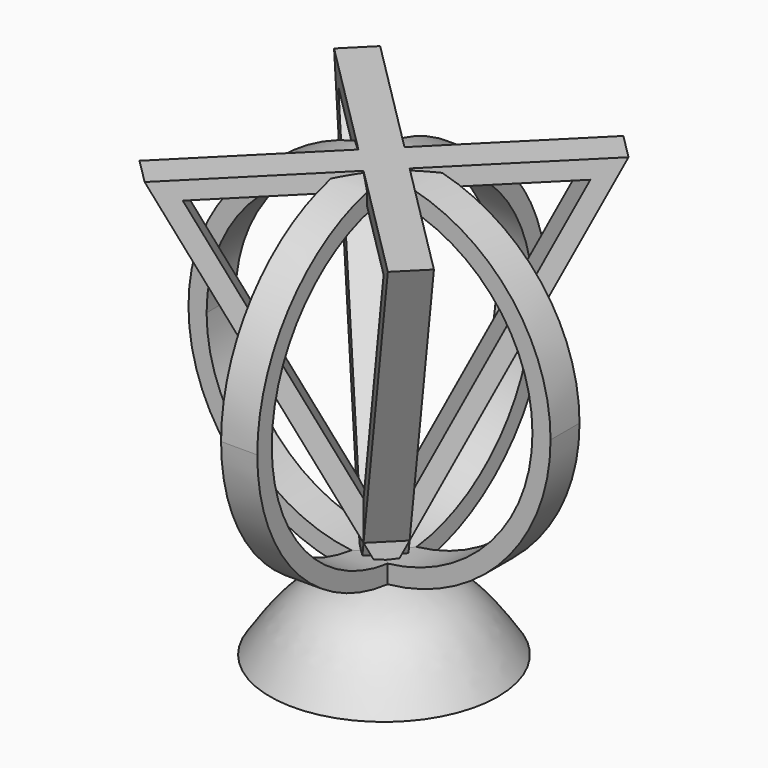
from build123d import *

# Parameters (mm, degrees)
F1_DEPTH = 5.08
F2_DEPTH = 5.08
F3_COUNT = 4
F6_DEPTH = 5.08
F7_DEPTH = 5.08
F8_COUNT = 4


with BuildPart() as f1:
    # F0 (on Front) → F1 (new body)
    with BuildSketch(Plane.XZ):
        with BuildLine():
            ThreePointArc((0, 45.72), (32.328922, 32.328922), (45.72, 0))
            ThreePointArc((45.72, 0), (32.328922, -32.328922), (0, -45.72))
            Line((0, -45.72), (0, -50.8))
            ThreePointArc((0, -50.8), (35.921024, -35.921024), (50.8, 0))
            ThreePointArc((50.8, 0), (35.921024, 35.921024), (0, 50.8))
            Line((0, 50.8), (0, 45.72))
        make_face()
    extrude(amount=F1_DEPTH)

    # F0 (on Front) → F2 (join)
    with BuildSketch(Plane.XZ):
        with BuildLine():
            ThreePointArc((0, 45.72), (32.328922, 32.328922), (45.72, 0))
            ThreePointArc((45.72, 0), (32.328922, -32.328922), (0, -45.72))
            Line((0, -45.72), (0, -50.8))
            ThreePointArc((0, -50.8), (35.921024, -35.921024), (50.8, 0))
            ThreePointArc((50.8, 0), (35.921024, 35.921024), (0, 50.8))
            Line((0, 50.8), (0, 45.72))
        make_face()
    extrude(amount=-F2_DEPTH)


with BuildPart() as f3_1:
    # F3: instance of F1
    add(f1.part.rotate(Axis((0, 0, -2.54), (0, 0, 1)), 1 * 360 / F3_COUNT))


with BuildPart() as f3_2:
    # F3: instance of F1
    add(f1.part.rotate(Axis((0, 0, -2.54), (0, 0, 1)), 2 * 360 / F3_COUNT))


with BuildPart() as f3_3:
    # F3: instance of F1
    add(f1.part.rotate(Axis((0, 0, -2.54), (0, 0, 1)), 3 * 360 / F3_COUNT))


with BuildPart() as f6:
    # F5 (on line) → F6 (new body)
    with BuildSketch(Plane(origin=(0, 0, 0), x_dir=(-0.707107, -0.707107, 0), z_dir=(-0.707107, 0.707107, 0))):
        Polygon((0, 45.72), (0, 50.8), (-53.34, 50.8), (0, -50.8), (0, -39.871365), (-44.935466, 45.72), align=None)
    extrude(amount=F6_DEPTH)


with BuildPart() as f7:
    # F7 (new): a face of the model
    f7_faces = [f6.part.faces().sort_by_distance(p)[0] for p in [
        (15.887086, 15.887086, 46.867506),
    ]]
    extrude(f7_faces, amount=F7_DEPTH)


with BuildPart() as f8_1:
    # F8: instance of F7
    add(f7.part.rotate(Axis((0, 0, -2.54), (0, 0, 1)), 1 * 360 / F8_COUNT))


with BuildPart() as f8_2:
    # F8: instance of F7
    add(f7.part.rotate(Axis((0, 0, -2.54), (0, 0, 1)), 2 * 360 / F8_COUNT))


with BuildPart() as f8_3:
    # F8: instance of F7
    add(f7.part.rotate(Axis((0, 0, -2.54), (0, 0, 1)), 3 * 360 / F8_COUNT))


with BuildPart() as f8_4:
    # F8: instance of F6
    add(f6.part.rotate(Axis((0, 0, -2.54), (0, 0, 1)), 1 * 360 / F8_COUNT))


with BuildPart() as f8_5:
    # F8: instance of F6
    add(f6.part.rotate(Axis((0, 0, -2.54), (0, 0, 1)), 2 * 360 / F8_COUNT))


with BuildPart() as f8_6:
    # F8: instance of F6
    add(f6.part.rotate(Axis((0, 0, -2.54), (0, 0, 1)), 3 * 360 / F8_COUNT))


with BuildPart() as f10:
    # F9 (on Front) → F10 (revolve)
    with BuildSketch(Plane.XZ):
        with BuildLine():
            Line((5.356453, -50.8), (0, -50.8))
            Line((0, -50.8), (0, -71.626157))
            Line((0, -71.626157), (31.985845, -71.626157))
            add(Edge.make_bspline(
                [(5.356453, -50.8), (10.334263, -52.157935), (20.921177, -55.046021), (28.153862, -65.884023), (31.985845, -71.626157)],
                knots=[0, 0, 0, 0, 0.470185, 1, 1, 1, 1], degree=3))
        make_face()
    revolve(axis=Axis((0, 0, -61.213078), (0, 0, -1)))


with BuildPart() as f3_1_1:
    add(f3_1.part)

    # F11: union F8_1, F8_4, F8_2, F8_5, F3_3, F8_3, F10, F1, F7, F6, F8_6, F3_2
    add(f8_1.part)
    add(f8_4.part)
    add(f8_2.part)
    add(f8_5.part)
    add(f3_3.part)
    add(f8_3.part)
    add(f10.part)
    add(f1.part)
    add(f7.part)
    add(f6.part)
    add(f8_6.part)
    add(f3_2.part)


solid = f3_1_1.part
